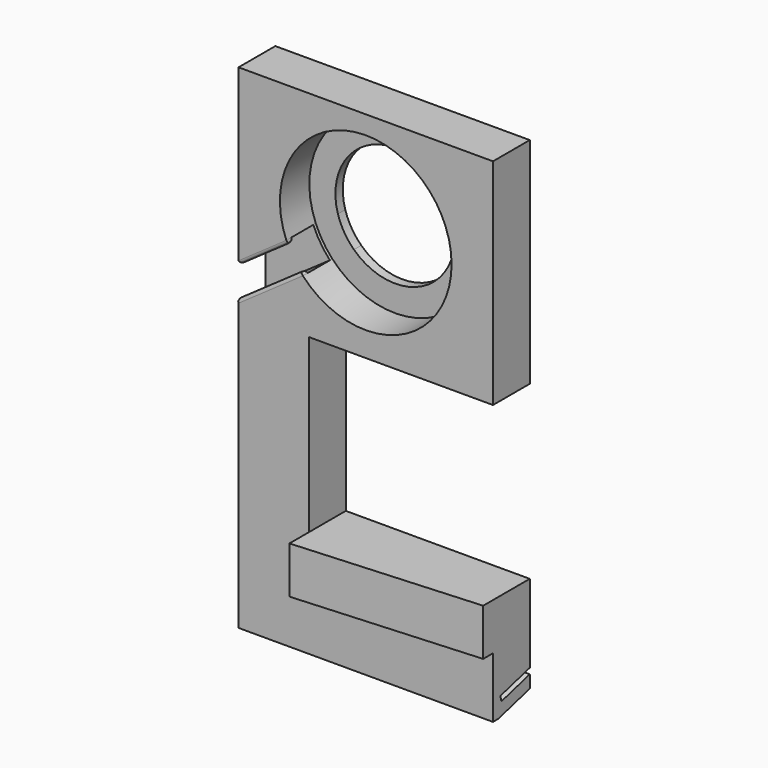
from build123d import *

# Parameters (mm, degrees)
F1_DEPTH  = 7.5
F2_DEPTH  = 1.5
F3_DEPTH  = 2
F5_DEPTH  = 45
F6_DEPTH  = 45
F7_W      = 9.5182569801
F7_H      = 1
F8_DEPTH  = 0.5
F9_W      = 12.8092049275
F9_H      = 1
F10_DEPTH = 0.5
F11_R     = 0.49999
F12_R     = 0.49999
F13_W     = 30
F13_H     = 7.6395883262
F14_DEPTH = 11.5
F16_DEPTH = 12.5


# Not quite as in the source:
# - a fillet or chamfer is up to 0.001 mm smaller than in the source, because OpenCascade refuses the exact size


with BuildPart() as f1:
    # F0 (on Front) → F1 (new body)
    with BuildSketch(Plane.XZ):
        with BuildLine():
            Line((-20.75, -40.25), (20.75, -40.25))
            Line((20.75, -40.25), (20.75, -22.75))
            Line((20.75, -22.75), (-9.25, -22.75))
            Line((-9.25, -22.75), (-9.25, 5.25))
            Line((-9.25, 5.25), (20.75, 5.25))
            Line((20.75, 5.25), (20.75, 40.25))
            Line((20.75, 40.25), (-20.75, 40.25))
            Line((-20.75, 40.25), (-20.75, 12.4785664195))
            Line((-20.75, 12.4785664195), (-12.9531003366, 17.9380143384))
            ThreePointArc((-12.9531003366, 17.9380143384), (-2.707082866, 36.9857818255), (14, 23.25))
            ThreePointArc((14, 23.25), (5.1184768061, 10.2192212364), (-10.2573135979, 13.7217515905))
            Line((-10.2573135979, 13.7217515905), (-20.75, 6.3746934757))
            Line((-20.75, 6.3746934757), (-20.75, -40.25))
        make_face()
    extrude(amount=F1_DEPTH)

    # F0 (on Front) → F2 (join)
    with BuildSketch(Plane.XZ):
        with BuildLine():
            ThreePointArc((-12.9531003366, 17.9380143384), (-11.7951280893, 15.7084515279), (-10.2573135979, 13.7217515905))
            Line((-10.2573135979, 13.7217515905), (-6.7277993643, 16.1931440631))
            ThreePointArc((-6.7277993643, 16.1931440631), (-8.3148780488, 18.158310395), (-9.3438531565, 20.4652364212))
            Line((-9.3438531565, 20.4652364212), (-12.9531003366, 17.9380143384))
        make_face()
        with BuildLine():
            Line((-6.7277993643, 16.1931440631), (-10.2573135979, 13.7217515905))
            ThreePointArc((-10.2573135979, 13.7217515905), (5.1184768061, 10.2192212364), (14, 23.25))
            ThreePointArc((14, 23.25), (-2.707082866, 36.9857818255), (-12.9531003366, 17.9380143384))
            Line((-12.9531003366, 17.9380143384), (-9.3438531565, 20.4652364212))
            ThreePointArc((-9.3438531565, 20.4652364212), (-1.4071125975, 32.8979290077), (9.75, 23.25))
            ThreePointArc((9.75, 23.25), (3.8383887374, 14.2873401325), (-6.7277993643, 16.1931440631))
        make_face()
    extrude(amount=F2_DEPTH)

    # F0 (on Front) → F3 (join)
    with BuildSketch(Plane.XZ):
        with BuildLine():
            Line((-20.75, 12.4785664195), (-20.75, 6.3746934757))
            Line((-20.75, 6.3746934757), (-10.2573135979, 13.7217515905))
            ThreePointArc((-10.2573135979, 13.7217515905), (-11.7951280893, 15.7084515279), (-12.9531003366, 17.9380143384))
            Line((-12.9531003366, 17.9380143384), (-20.75, 12.4785664195))
        make_face()
    extrude(amount=F3_DEPTH)

    # F4 (on face) → F5 (cut)
    with BuildSketch(Plane.YZ.offset(20.75)):
        Polygon((-6.4365309663, -40.25), (0, -40.25), (0, -38.5253367255), align=None)
    extrude(amount=-F5_DEPTH, mode=Mode.SUBTRACT)

    # F4 (on face) → F6 (cut)
    with BuildSketch(Plane.YZ.offset(20.75)):
        Polygon((-5.7670628594, -38.0000642006), (0, -36.4547843647), (0, -35.5230358023), (-6, -37.1307309569), align=None)
    extrude(amount=-F6_DEPTH, mode=Mode.SUBTRACT)

    # F7 (on face) → F8 (join)
    with BuildSketch(Plane(origin=(-12.6895494042, 0, 18.122554688), x_dir=(0.8191520443, 0, 0.5735764364), z_dir=(0.5735764364, 0, -0.8191520443))):
        with Locations((-5.0808647713, 7)):
            Rectangle(F7_W, F7_H)
    extrude(amount=F8_DEPTH)

    # F9 (on face) → F10 (join)
    with BuildSketch(Plane(origin=(-9.8216672224, 0, 14.0267944666), x_dir=(0.8191520443, 0, 0.5735764364), z_dir=(-0.5735764364, 0, 0.8191520443))):
        with Locations((-6.9364284886, -7)):
            Rectangle(F9_W, F9_H)
    extrude(amount=F10_DEPTH)

    # F11 (radius 0.5 in the source; OpenCascade refuses exactly that, so slightly less here)
    f11_edges = [f1.edges().sort_by_distance(p)[0] for p in [
        (-20.463212, -7, 12.06899),
        (-16.564762, -6.5, 14.798714),
        (-12.666312, -7, 17.528438),
        (-16.564762, -7.5, 14.798714),
    ]]
    fillet(f11_edges, radius=F11_R)

    # F12 (radius 0.5 in the source; OpenCascade refuses exactly that, so slightly less here)
    f12_edges = [f1.edges().sort_by_distance(p)[0] for p in [
        (-15.790445, -6.5, 10.457799),
        (-21.036788, -7, 6.784269),
        (-15.790445, -7.5, 10.457799),
        (-10.544102, -7, 14.131328),
    ]]
    fillet(f12_edges, radius=F12_R)

    # F13 (on face) → F14 (join)
    with BuildSketch(Plane(origin=(0, 0, 0), x_dir=(-1, 0, 0), z_dir=(0, 1, 0))):
        with Locations((-5.75, -26.5697941631)):
            Rectangle(F13_W, F13_H)
    extrude(amount=-F14_DEPTH)

    # F15 (on face) → F16 (cut, symmetric)
    with BuildSketch(Plane(origin=(0, 0, -30.3895883262), x_dir=(1, 0, 0), z_dir=(0, 0, -1))):
        Polygon((-9.25, 11.5), (20.75, 9.5), (20.75, 11.5), align=None)
    extrude(amount=F16_DEPTH, both=True, mode=Mode.SUBTRACT)


solid = f1.part
